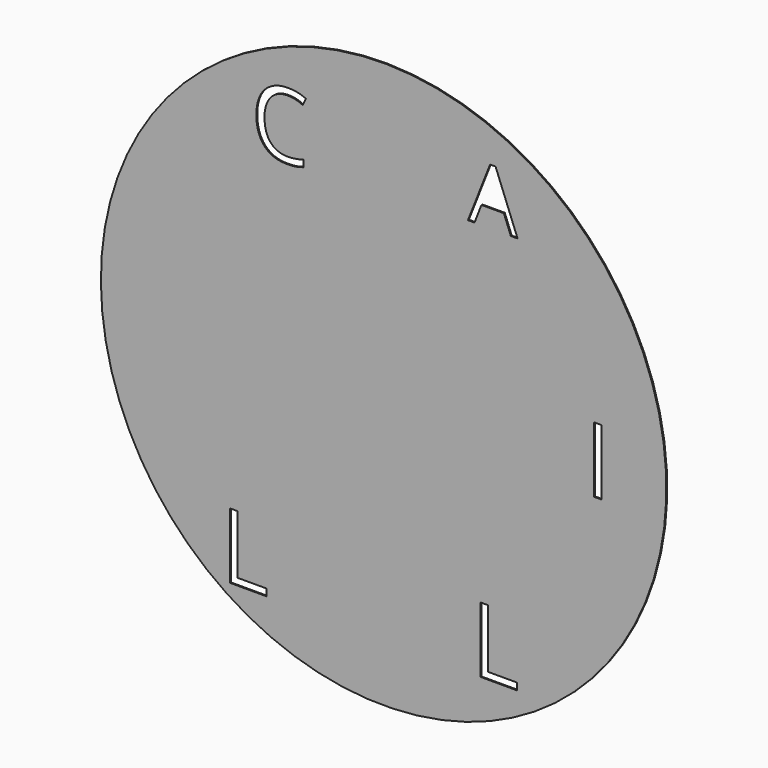
from build123d import *

# Parameters (mm, degrees)
F0_W         = 32.196484375
F0_H         = 277.0352864583
F0_R         = 52.451
F0_TEXT_SIZE = 388.0555555556
F1_DEPTH     = 4.76


# Not quite as in the source:
# - Text() gives the source's letters only with a copy of the font that has no kerning and outlines rounded to 1/6400 em; it was checked with that copy


with BuildPart() as f1:
    # F0 (on Front) → F1 (new body)
    with BuildSketch(Plane.XZ):
        with BuildLine():
            ThreePointArc((2158.8500577526, 874.1527002855), (2258.4775336104, 1140.4086406168), (2292.3265282944, 1422.6711164552))
            ThreePointArc((2292.3265282944, 1422.6711164552), (2252.5213155869, 1728.3743563817), (2135.7601505065, 2013.6912962738))
            ThreePointArc((2135.7601505065, 2013.6912962738), (1707.8041447602, 2449.2865391299), (1120.431996217, 2616.2701238589))
            ThreePointArc((1120.431996217, 2616.2701238589), (546.8171320189, 2481.3378166311), (107.626605235, 2088.4607097058))
            ThreePointArc((107.626605235, 2088.4607097058), (-88.708434548, 1547.697445701), (-9.3253919009, 977.8986320098))
            ThreePointArc((-9.3253919009, 977.8986320098), (420.4074393623, 440.167711257), (1075.5956769647, 229.0913679434))
            ThreePointArc((1075.5956769647, 229.0913679434), (1709.3226667722, 396.9584289931), (2158.8500577526, 874.1527002855))
        make_face()
        with BuildLine():
            ThreePointArc((1321.1423108478, 469.9659194545), (1248.9347207072, 297.982127357), (1075.5956769647, 229.0913679434))
            ThreePointArc((1075.5956769647, 229.0913679434), (911.5119009883, 641.949711552), (1321.1423108478, 469.9659194545))
        make_face(mode=Mode.SUBTRACT)
        Polygon((603.7878659405, 473.4311741282), (449.3538815655, 473.4311741282), (449.3538815655, 750.4664605866), (481.5503659405, 750.4664605866), (481.5503659405, 502.5959744755), (603.7878659405, 502.5959744755), align=None, mode=Mode.SUBTRACT)
        with BuildLine():
            ThreePointArc((455.167557139, 1067.6574971527), (259.9582515826, 831.1145023402), (-9.3253919009, 977.8986320098))
            ThreePointArc((-9.3253919009, 977.8986320098), (168.5388626953, 1304.2004919652), (455.167557139, 1067.6574971527))
        make_face(mode=Mode.SUBTRACT)
        Polygon((1661.7239450011, 467.7944920779), (1507.2899606261, 467.7944920779), (1507.2899606261, 744.8297785362), (1539.4864450011, 744.8297785362), (1539.4864450011, 496.9592924251), (1661.7239450011, 496.9592924251), align=None, mode=Mode.SUBTRACT)
        with BuildLine():
            ThreePointArc((2185.7867414475, 984.8483771193), (2178.9557272807, 927.8854115229), (2158.8500577526, 874.1527002855))
            ThreePointArc((2158.8500577526, 874.1527002855), (1710.7797556142, 1041.8113427157), (2185.7867414475, 984.8483771193))
        make_face(mode=Mode.SUBTRACT)
        Polygon((248.4161892361, 1654.7829805245), (248.4161892361, 1377.7476940661), (216.2197048611, 1377.7476940661), (216.2197048611, 1508.1101072606), (70.2744357639, 1508.1101072606), (70.2744357639, 1377.7476940661), (38.0779513889, 1377.7476940661), (38.0779513889, 1654.7829805245), (70.2744357639, 1654.7829805245), (70.2744357639, 1536.9111055245), (216.2197048611, 1536.9111055245), (216.2197048611, 1654.7829805245), align=None, mode=Mode.SUBTRACT)
        with BuildLine():
            ThreePointArc((548.5176482659, 1954.0987114807), (237.3672452968, 1723.6436950502), (107.626605235, 2088.4607097058))
            ThreePointArc((107.626605235, 2088.4607097058), (377.830051235, 2184.5537279113), (548.5176482659, 1954.0987114807))
        make_face(mode=Mode.SUBTRACT)
        with BuildLine():
            add(Edge.make_bspline(
                [(757.0453405304, 2349.3687452396), (725.576460322, 2364.1027296146), (694.1075801137, 2364.1027296146)],
                knots=[0, 0, 0, 1, 1, 1], degree=2))
            add(Edge.make_bspline(
                [(694.1075801137, 2364.1027296146), (648.4504186554, 2364.1027296146), (622.0141339331, 2333.694938816)],
                knots=[0, 0, 0, 1, 1, 1], degree=2))
            add(Edge.make_bspline(
                [(622.0141339331, 2333.694938816), (595.5778492109, 2303.2871480174), (595.5778492109, 2250.414578573)],
                knots=[0, 0, 0, 1, 1, 1], degree=2))
            add(Edge.make_bspline(
                [(595.5778492109, 2250.414578573), (595.5778492109, 2196.0868007952), (621.0743118845, 2166.4066141632)],
                knots=[0, 0, 0, 1, 1, 1], degree=2))
            add(Edge.make_bspline(
                [(621.0743118845, 2166.4066141632), (646.5707745581, 2136.7264275313), (693.7437780304, 2136.7264275313)],
                knots=[0, 0, 0, 1, 1, 1], degree=2))
            add(Edge.make_bspline(
                [(693.7437780304, 2136.7264275313), (722.7266773359, 2136.7264275313), (759.8951235165, 2147.1554205868)],
                knots=[0, 0, 0, 1, 1, 1], degree=2))
            Line((759.8951235165, 2147.1554205868), (759.8951235165, 2118.9607591285))
            add(Edge.make_bspline(
                [(759.8951235165, 2118.9607591285), (731.0941252526, 2108.1073303091), (688.8324499054, 2108.1073303091)],
                knots=[0, 0, 0, 1, 1, 1], degree=2))
            add(Edge.make_bspline(
                [(688.8324499054, 2108.1073303091), (627.6530662248, 2108.1073303091), (594.3954924401, 2145.2757764896)],
                knots=[0, 0, 0, 1, 1, 1], degree=2))
            add(Edge.make_bspline(
                [(594.3954924401, 2145.2757764896), (561.1379186554, 2182.4442226702), (561.1379186554, 2250.8390143368)],
                knots=[0, 0, 0, 1, 1, 1], degree=2))
            add(Edge.make_bspline(
                [(561.1379186554, 2250.8390143368), (561.1379186554, 2293.6463928091), (577.145210322, 2325.8428771841)],
                knots=[0, 0, 0, 1, 1, 1], degree=2))
            add(Edge.make_bspline(
                [(577.145210322, 2325.8428771841), (593.1525019887, 2358.0393615591), (623.3783917456, 2375.4715447188)],
                knots=[0, 0, 0, 1, 1, 1], degree=2))
            add(Edge.make_bspline(
                [(623.3783917456, 2375.4715447188), (653.6042815026, 2392.9037278785), (694.5320158776, 2392.9037278785)],
                knots=[0, 0, 0, 1, 1, 1], degree=2))
            add(Edge.make_bspline(
                [(694.5320158776, 2392.9037278785), (738.0669985165, 2392.9037278785), (770.6879186554, 2377.017703573)],
                knots=[0, 0, 0, 1, 1, 1], degree=2))
            Line((770.6879186554, 2377.017703573), (757.0453405304, 2349.3687452396))
        make_face(mode=Mode.SUBTRACT)
        Polygon((1232.5119970856, 1346.8144421461), (978.6425102177, 1338.6729657801), (1098.5265282944, 1562.6011288364), align=None, mode=Mode.SUBTRACT)
        with Locations((2003.1159791226, 1431.6180757572)):
            Rectangle(F0_W, F0_H, mode=Mode.SUBTRACT)
        with BuildLine():
            ThreePointArc((2167.3565745389, 1894.4184001434), (1693.5516043298, 1832.7248879987), (2135.7601505065, 2013.6912962738))
            ThreePointArc((2135.7601505065, 2013.6912962738), (2159.3235447481, 1956.111912288), (2167.3565745389, 1894.4184001434))
        make_face(mode=Mode.SUBTRACT)
        Polygon((1664.0469826933, 2148.1028804173), (1635.5906561509, 2148.1028804173), (1606.1512928734, 2223.2793212648), (1511.4175948749, 2223.2793212648), (1482.3404030261, 2148.1028804173), (1454.50494179, 2148.1028804173), (1547.9451704002, 2385.4803825566), (1571.0724030629, 2385.4803825566), align=None, mode=Mode.SUBTRACT)
        with BuildLine():
            ThreePointArc((1356.9302942734, 2375.3916857301), (944.0999862501, 2206.606417609), (1120.431996217, 2616.2701238589))
            ThreePointArc((1120.431996217, 2616.2701238589), (1287.9226022967, 2544.1769538513), (1356.9302942734, 2375.3916857301))
        make_face(mode=Mode.SUBTRACT)
        with BuildLine():
            ThreePointArc((548.5176482659, 1954.0987114807), (377.830051235, 2184.5537279113), (107.626605235, 2088.4607097058))
            ThreePointArc((107.626605235, 2088.4607097058), (237.3672452968, 1723.6436950502), (548.5176482659, 1954.0987114807))
        make_face()
        with BuildLine():
            ThreePointArc((455.167557139, 1067.6574971527), (168.5388626953, 1304.2004919652), (-9.3253919009, 977.8986320098))
            ThreePointArc((-9.3253919009, 977.8986320098), (259.9582515826, 831.1145023402), (455.167557139, 1067.6574971527))
        make_face()
        with BuildLine():
            ThreePointArc((1321.1423108478, 469.9659194545), (911.5119009883, 641.949711552), (1075.5956769647, 229.0913679434))
            ThreePointArc((1075.5956769647, 229.0913679434), (1248.9347207072, 297.982127357), (1321.1423108478, 469.9659194545))
        make_face()
        with BuildLine():
            ThreePointArc((1356.9302942734, 2375.3916857301), (1287.9226022967, 2544.1769538513), (1120.431996217, 2616.2701238589))
            ThreePointArc((1120.431996217, 2616.2701238589), (944.0999862501, 2206.606417609), (1356.9302942734, 2375.3916857301))
        make_face()
        with BuildLine():
            ThreePointArc((2167.3565745389, 1894.4184001434), (2159.3235447481, 1956.111912288), (2135.7601505065, 2013.6912962738))
            ThreePointArc((2135.7601505065, 2013.6912962738), (1693.5516043298, 1832.7248879987), (2167.3565745389, 1894.4184001434))
        make_face()
        with BuildLine():
            ThreePointArc((2185.7867414475, 984.8483771193), (1710.7797556142, 1041.8113427157), (2158.8500577526, 874.1527002855))
            ThreePointArc((2158.8500577526, 874.1527002855), (2178.9557272807, 927.8854115229), (2185.7867414475, 984.8483771193))
        make_face()
        Polygon((1098.5265282944, 1562.6011288364), (978.6425102177, 1338.6729657801), (1232.5119970856, 1346.8144421461), align=None)
        with Locations((1098.5265282944, 1422.6711164552)):
            Circle(F0_R, mode=Mode.SUBTRACT)
        with Locations((0, 1377.7476940661)):
            Text('H', F0_TEXT_SIZE, font='Open Sans', text_align=(TextAlign.LEFT, TextAlign.BOTTOM))
        with Locations((1098.5265282944, 1422.6711164552)):
            Circle(F0_R)
    extrude(amount=F1_DEPTH)


solid = f1.part
